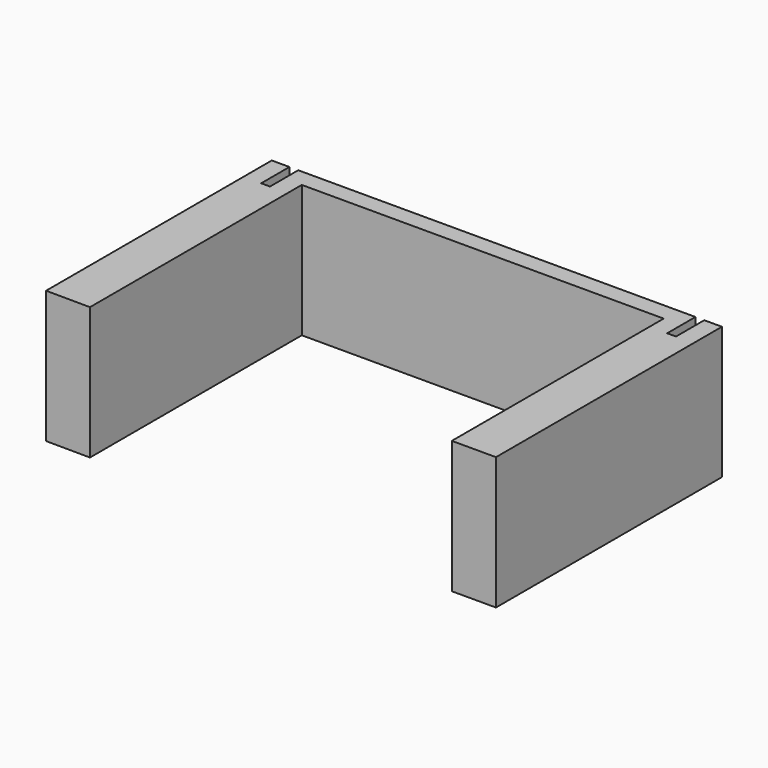
from build123d import *

# Parameters (mm, degrees)
F1_DEPTH = 15


# Not quite as in the source:
# - a feature names something its author has since deleted; it is built from what else it names


with BuildPart() as f1:
    # F0 (on Top) → F1 (new body)
    with BuildSketch(Plane.XY):
        Polygon((-21.2294230163, -33.7162413895), (-21.2294230163, -3.7162413895), (19.7705769837, -3.7162413895), (19.7705769837, -33.7162413895), (24.7705769837, -33.7162413895), (24.7705769837, -1.7162413895), (22.7705769837, -1.7162413895), (22.7705769837, -5.7162413895), (21.7705769837, -5.7162413895), (21.7705769837, -1.7162413895), (-23.2294230163, -1.7162413895), (-23.2294230163, -5.7162413895), (-24.2294230163, -5.7162413895), (-24.2294230163, -1.7162413895), (-26.2294230163, -1.7162413895), (-26.2294230163, -33.6776562035), align=None)
    extrude(amount=F1_DEPTH)


solid = f1.part
